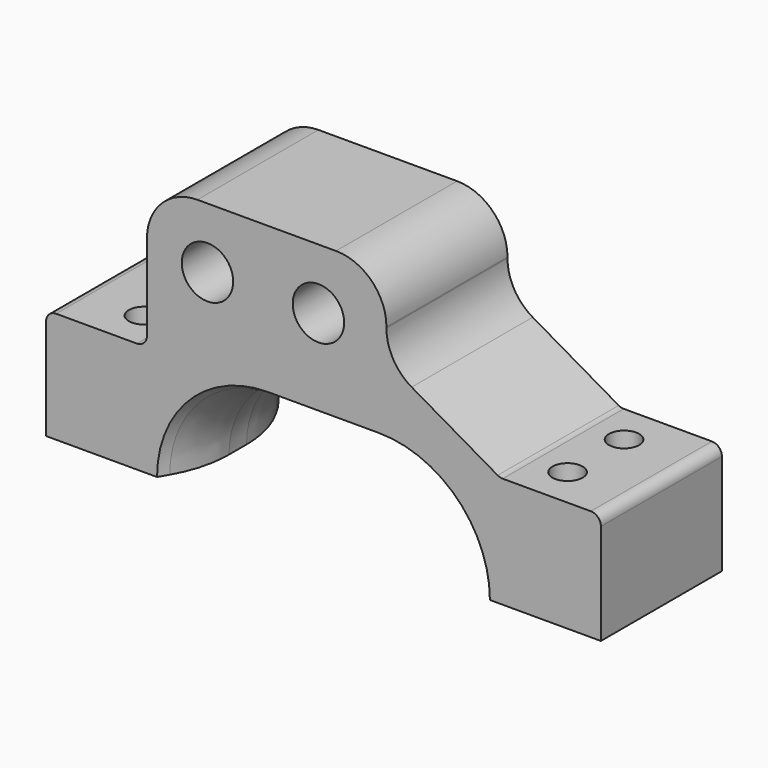
from build123d import *

# Parameters (mm, degrees)
F0_R       = 2.55
F1_DEPTH   = 15
F2_R       = 4.99999
F3_R       = 1.5
F4_DEPTH   = 25
F5_R       = 1.5
F6_DEPTH   = 25
F7_SIZE2   = 3.4641016151
F7_SIZE    = 2
F7_2_SIZE2 = 3.4641016151
F7_2_SIZE  = 2
F8_R       = 11
F9_R       = 1
F10_W      = 76.274741441
F10_H      = 34.1036086902
F11_DEPTH  = 25
F12_W      = 2
F12_H      = 11
F13_DEPTH  = 15
F14_R      = 1


# Not quite as in the source:
# - a fillet or chamfer is up to 0.001 mm smaller than in the source, because OpenCascade refuses the exact size


with BuildPart() as f1:
    # F0 (on Front) → F1 (new body)
    with BuildSketch(Plane.XZ):
        Polygon((-20, 11), (-20, 0), (-20, -10), (-12, -10), (-12, -15), (23, -15), (23, -10), (31, -10), (31, 11), (23, 11), (11.7416697508, 17.5), (11.7416697508, 25.5), (-12, 25.5), (-12, 11), align=None)
        with BuildLine():
            ThreePointArc((0, -9), (-9, 0), (0, 9))
            Line((0, 9), (11, 9))
            ThreePointArc((11, 9), (20, 0), (11, -9))
            Line((11, -9), (0, -9))
        make_face(mode=Mode.SUBTRACT)
        with Locations((-6, 19.5)):
            Circle(F0_R, mode=Mode.SUBTRACT)
        with Locations((5, 19.5)):
            Circle(F0_R, mode=Mode.SUBTRACT)
    extrude(amount=F1_DEPTH)

    # F2 (radius 5 in the source; OpenCascade refuses exactly that, so slightly less here)
    f2_edges = [f1.edges().sort_by_distance(p)[0] for p in [
        (11.74167, -7.5, 25.5),
        (-12, -7.5, 25.5),
        (-12, -7.5, -15),
        (23, -7.5, -15),
        (11.74167, -7.5, 17.5),
    ]]
    fillet(f2_edges, radius=F2_R)

    # F3 (on face) → F4 (cut)
    with BuildSketch(Plane.XY.offset(11)):
        with Locations((-15.5, -4)):
            Circle(F3_R)
        with Locations((-15.5, -11)):
            Circle(F3_R)
    extrude(amount=-F4_DEPTH, mode=Mode.SUBTRACT)

    # F5 (on face) → F6 (cut)
    with BuildSketch(Plane.XY.offset(11)):
        with Locations((26.5, -4)):
            Circle(F5_R)
        with Locations((26.5, -11)):
            Circle(F5_R)
    extrude(amount=-F6_DEPTH, mode=Mode.SUBTRACT)

    # F7
    f7_edges = [f1.edges().sort_by_distance(p)[0] for p in [
        (-9, 0, 0),
        (5.5, 0, 9),
    ]]
    f7_side = f1.faces().sort_by_distance((11.090421, 0, 20.443378))[0]
    chamfer(f7_edges, length=F7_SIZE, length2=F7_SIZE2, reference=f7_side)

    # F7#2
    f7_2_edges = [f1.edges().sort_by_distance(p)[0] for p in [
        (5.5, -15, 9),
    ]]
    f7_2_side = f1.faces().sort_by_distance((11.090421, -15, 20.443378))[0]
    chamfer(f7_2_edges, length=F7_2_SIZE, length2=F7_2_SIZE2, reference=f7_2_side)

    # F8
    f8_edges = [f1.edges().sort_by_distance(p)[0] for p in [
        (-9, -11.535898, 0),
        (-9, -3.464102, 0),
        (5.5, -11.535898, 9),
        (5.5, -3.464102, 9),
    ]]
    fillet(f8_edges, radius=F8_R)

    # F9
    f9_edges = [f1.edges().sort_by_distance(p)[0] for p in [
        (-12, -7.5, 11),
        (23, -7.5, 11),
    ]]
    fillet(f9_edges, radius=F9_R)

    # F10 (on Top) → F11 (cut)
    with BuildSketch(Plane.XY):
        with Locations((3.48370336, -7.8841676004)):
            Rectangle(F10_W, F10_H)
    extrude(amount=-F11_DEPTH, mode=Mode.SUBTRACT)

    # F12 (on face) → F13 (join)
    with BuildSketch(Plane.XZ.offset(15)):
        with Locations((-21, 5.5)):
            Rectangle(F12_W, F12_H)
        with Locations((32, 5.5)):
            Rectangle(F12_W, F12_H)
    extrude(amount=-F13_DEPTH)

    # F14
    f14_edges = [f1.edges().sort_by_distance(p)[0] for p in [
        (-22, -7.5, 11),
        (33, -7.5, 11),
    ]]
    fillet(f14_edges, radius=F14_R)


solid = f1.part
